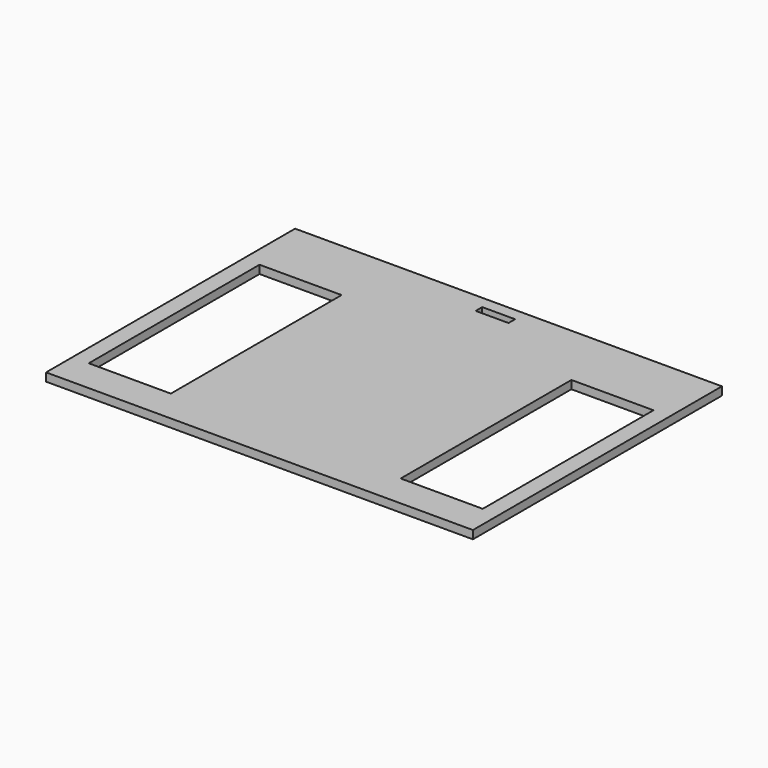
from build123d import *

# Parameters (mm, degrees)
F0_W     = 12.7
F0_H     = 3.175
F1_DEPTH = 3.175


# Not quite as in the source:
# - a feature names something its author has since deleted; it is built from what else it names


with BuildPart() as f1:
    # F0 (on Top) → F1 (new body)
    with BuildSketch(Plane.XY):
        Polygon((0, -12.7), (0, -120.396), (6.35, -120.396), (6.35, -37.846), (38.1, -37.846), (38.1, -120.396), (127, -120.396), (127, -37.846), (158.75, -37.846), (158.75, -120.396), (165.1, -120.396), (165.1, -12.7), align=None)
        with Locations((82.55, -19.05)):
            Rectangle(F0_W, F0_H, mode=Mode.SUBTRACT)
        Polygon((6.35, -120.396), (0, -120.396), (0, -133.096), (165.1, -133.096), (165.1, -120.396), (158.75, -120.396), (127, -120.396), (38.1, -120.396), align=None)
    extrude(amount=F1_DEPTH)


solid = f1.part
